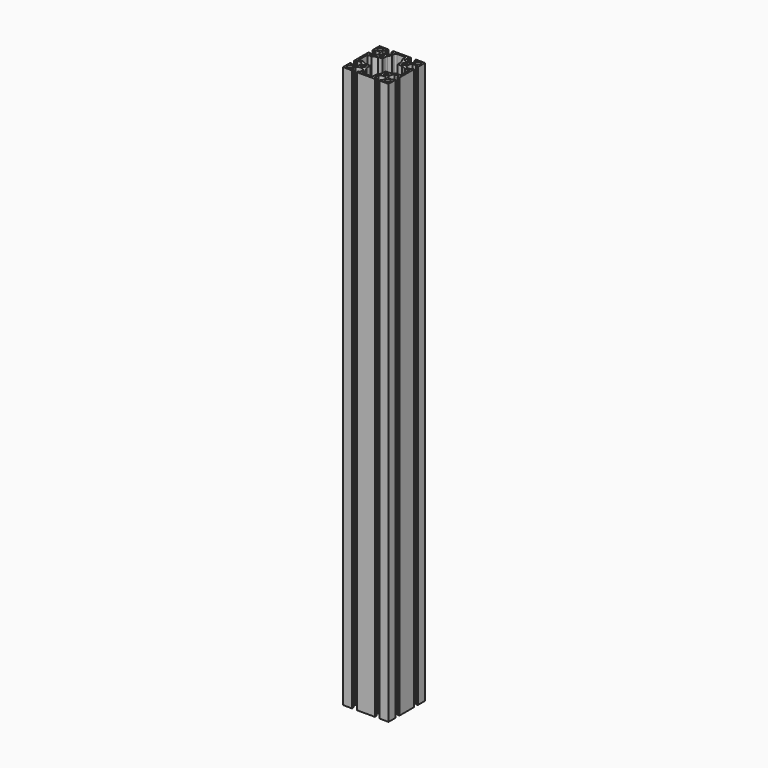
from build123d import *

# Parameters (mm, degrees)
F0_R     = 3
F0_R_2   = 2.5
F1_DEPTH = 740
F2_R     = 2
F3_R     = 7


# Not quite as in the source:
# - a feature names something its author has since deleted; it is built from what else it names


with BuildPart() as f1:
    # F0 (on Top) → F1 (new body)
    with BuildSketch(Plane.XY):
        with BuildLine():
            Line((18.15, -30), (30, -30))
            Line((30, -30), (30, -18.15))
            Line((30, -18.15), (27.5, -18.15))
            Line((27.5, -18.15), (27.5, -20.15))
            Line((27.5, -20.15), (21.5477069044, -20.15))
            ThreePointArc((21.5477069044, -20.15), (19.5, -15), (21.5477069044, -9.85))
            Line((21.5477069044, -9.85), (27.5, -9.85))
            Line((27.5, -9.85), (27.5, -11.85))
            Line((27.5, -11.85), (30, -11.85))
            Line((30, -11.85), (30, 11.85))
            Line((30, 11.85), (27.5, 11.85))
            Line((27.5, 11.85), (27.5, 9.85))
            Line((27.5, 9.85), (21.5477069044, 9.85))
            ThreePointArc((21.5477069044, 9.85), (19.5, 15), (21.5477069044, 20.15))
            Line((21.5477069044, 20.15), (27.5, 20.15))
            Line((27.5, 20.15), (27.5, 18.15))
            Line((27.5, 18.15), (30, 18.15))
            Line((30, 18.15), (30, 30))
            Line((30, 30), (18.15, 30))
            Line((18.15, 30), (18.15, 27.5))
            Line((18.15, 27.5), (20.15, 27.5))
            Line((20.15, 27.5), (20.15, 21.5477069044))
            ThreePointArc((20.15, 21.5477069044), (15, 19.5), (9.85, 21.5477069044))
            Line((9.85, 21.5477069044), (9.85, 27.5))
            Line((9.85, 27.5), (11.85, 27.5))
            Line((11.85, 27.5), (11.85, 30))
            Line((11.85, 30), (-11.85, 30))
            Line((-11.85, 30), (-11.85, 27.5))
            Line((-11.85, 27.5), (-9.85, 27.5))
            Line((-9.85, 27.5), (-9.85, 21.5477069044))
            ThreePointArc((-9.85, 21.5477069044), (-15, 19.5), (-20.15, 21.5477069044))
            Line((-20.15, 21.5477069044), (-20.15, 27.5))
            Line((-20.15, 27.5), (-18.15, 27.5))
            Line((-18.15, 27.5), (-18.15, 30))
            Line((-18.15, 30), (-30, 30))
            Line((-30, 30), (-30, 18.15))
            Line((-30, 18.15), (-27.5, 18.15))
            Line((-27.5, 18.15), (-27.5, 20.15))
            Line((-27.5, 20.15), (-21.5477069044, 20.15))
            ThreePointArc((-21.5477069044, 20.15), (-19.5, 15), (-21.5477069044, 9.85))
            Line((-21.5477069044, 9.85), (-27.5, 9.85))
            Line((-27.5, 9.85), (-27.5, 11.85))
            Line((-27.5, 11.85), (-30, 11.85))
            Line((-30, 11.85), (-30, -11.85))
            Line((-30, -11.85), (-27.5, -11.85))
            Line((-27.5, -11.85), (-27.5, -9.85))
            Line((-27.5, -9.85), (-21.5477069044, -9.85))
            ThreePointArc((-21.5477069044, -9.85), (-19.5, -15), (-21.5477069044, -20.15))
            Line((-21.5477069044, -20.15), (-27.5, -20.15))
            Line((-27.5, -20.15), (-27.5, -18.15))
            Line((-27.5, -18.15), (-30, -18.15))
            Line((-30, -18.15), (-30, -30))
            Line((-30, -30), (-18.15, -30))
            Line((-18.15, -30), (-18.15, -27.5))
            Line((-18.15, -27.5), (-20.15, -27.5))
            Line((-20.15, -27.5), (-20.15, -21.5477069044))
            ThreePointArc((-20.15, -21.5477069044), (-15, -19.5), (-9.85, -21.5477069044))
            Line((-9.85, -21.5477069044), (-9.85, -27.5))
            Line((-9.85, -27.5), (-11.85, -27.5))
            Line((-11.85, -27.5), (-11.85, -30))
            Line((-11.85, -30), (11.85, -30))
            Line((11.85, -30), (11.85, -27.5))
            Line((11.85, -27.5), (9.85, -27.5))
            Line((9.85, -27.5), (9.85, -21.5477069044))
            ThreePointArc((9.85, -21.5477069044), (15, -19.5), (20.15, -21.5477069044))
            Line((20.15, -21.5477069044), (20.15, -27.5))
            Line((20.15, -27.5), (18.15, -27.5))
            Line((18.15, -27.5), (18.15, -30))
        make_face()
        with Locations((-25, -25)):
            Circle(F0_R, mode=Mode.SUBTRACT)
        with Locations((-15, -15)):
            Circle(F0_R_2, mode=Mode.SUBTRACT)
        with Locations((25, -25)):
            Circle(F0_R, mode=Mode.SUBTRACT)
        with Locations((15, -15)):
            Circle(F0_R_2, mode=Mode.SUBTRACT)
        with Locations((-25, 25)):
            Circle(F0_R, mode=Mode.SUBTRACT)
        with Locations((-15, 15)):
            Circle(F0_R_2, mode=Mode.SUBTRACT)
        Polygon((-7, 22), (-7, 27.5), (0, 27.5), (7, 27.5), (7, 22), (10, 16), (10, 10), (16, 10), (22, 7), (27.5, 7), (27.5, 0), (27.5, -7), (22, -7), (16, -10), (10, -10), (10, -16), (7, -22), (7, -27.5), (0, -27.5), (-7, -27.5), (-7, -22), (-10, -16), (-10, -10), (-16, -10), (-22, -7), (-27.5, -7), (-27.5, 0), (-27.5, 7), (-22, 7), (-16, 10), (-10, 10), (-10, 16), align=None, mode=Mode.SUBTRACT)
        with Locations((15, 15)):
            Circle(F0_R_2, mode=Mode.SUBTRACT)
        with Locations((25, 25)):
            Circle(F0_R, mode=Mode.SUBTRACT)
    extrude(amount=F1_DEPTH)

    # F2
    f2_edges = [f1.edges().sort_by_distance(p)[0] for p in [
        (-7, 27.5, 370),
        (7, 27.5, 370),
    ]]
    fillet(f2_edges, radius=F2_R)

    # F3
    f3_edges = [f1.edges().sort_by_distance(p)[0] for p in [
        (-10, 16, 370),
        (10, 16, 370),
    ]]
    fillet(f3_edges, radius=F3_R)


solid = f1.part
